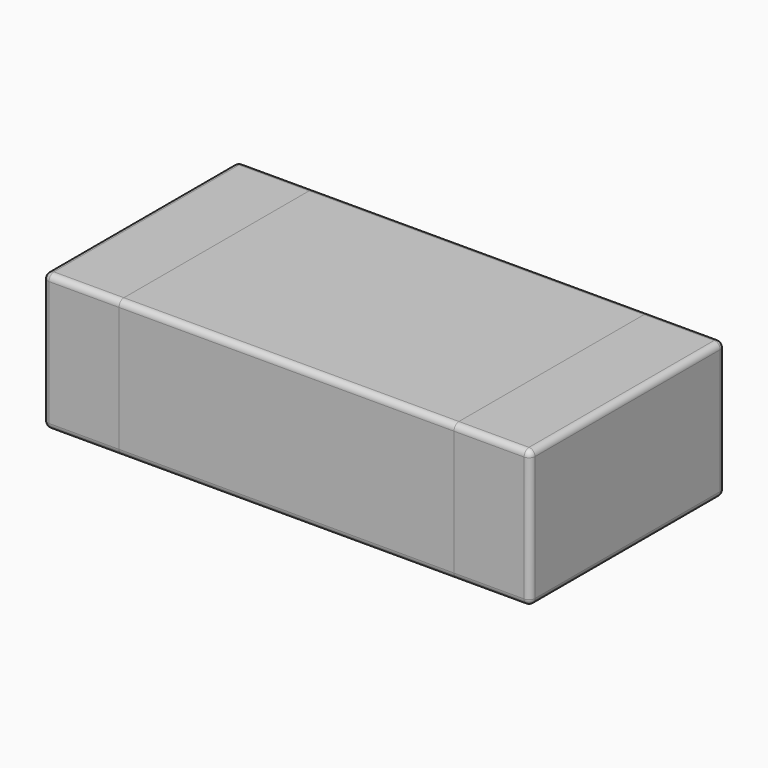
from build123d import *

# Parameters (mm, degrees)
F2_W     = 1.1
F2_H     = 0.8
F3_DEPTH = 0.43
F2_W_2   = 0.25
F4_DEPTH = 0.45
F5_DEPTH = 0.45
F6_DEPTH = 0.02
F7_R     = 0.01999
F7_2_R   = 0.01999
F7_3_R   = 0.01999
F7_4_R   = 0.01999


# Not quite as in the source:
# - a fillet or chamfer is up to 0.001 mm smaller than in the source, because OpenCascade refuses the exact size


with BuildPart() as f3:
    # F2 (on Top) → F3 (new body)
    with BuildSketch(Plane.XY):
        Rectangle(F2_W, F2_H)
    extrude(amount=F3_DEPTH)


with BuildPart() as f4:
    # F2 (on Top) → F4 (new body)
    with BuildSketch(Plane.XY):
        with Locations((-0.675, 0)):
            Rectangle(F2_W_2, F2_H)
    extrude(amount=F4_DEPTH)

    # F7 (radius 0.02 in the source; OpenCascade refuses exactly that, so slightly less here)
    f7_edges = [f4.edges().sort_by_distance(p)[0] for p in [
        (-0.675, -0.4, 0.45),
        (-0.8, 0.4, 0.225),
        (-0.8, -0.4, 0.225),
        (-0.8, 0, 0),
        (-0.8, 0, 0.45),
        (-0.675, 0.4, 0.45),
        (-0.675, 0.4, 0),
        (-0.675, -0.4, 0),
    ]]
    fillet(f7_edges, radius=F7_R)


with BuildPart() as f5:
    # F2 (on Top) → F5 (new body)
    with BuildSketch(Plane.XY):
        with Locations((0.675, 0)):
            Rectangle(F2_W_2, F2_H)
    extrude(amount=F5_DEPTH)

    # F7#2 (radius 0.02 in the source; OpenCascade refuses exactly that, so slightly less here)
    f7_2_edges = [f5.edges().sort_by_distance(p)[0] for p in [
        (0.675, -0.4, 0.45),
        (0.8, -0.4, 0.225),
        (0.8, 0.4, 0.225),
        (0.8, 0, 0),
        (0.8, 0, 0.45),
        (0.675, 0.4, 0.45),
        (0.675, 0.4, 0),
        (0.675, -0.4, 0),
    ]]
    fillet(f7_2_edges, radius=F7_2_R)


with BuildPart() as f6:
    # F6 (new): a face of the model
    f6_faces = [f3.part.faces().sort_by_distance(p)[0] for p in [
        (0, 0, 0.43),
    ]]
    extrude(f6_faces, amount=F6_DEPTH)

    # F7#4 (radius 0.02 in the source; OpenCascade refuses exactly that, so slightly less here)
    f7_4_edges = [f6.edges().sort_by_distance(p)[0] for p in [
        (0, -0.4, 0.45),
        (0, 0.4, 0.45),
    ]]
    fillet(f7_4_edges, radius=F7_4_R)


with BuildPart() as f3_1:
    add(f3.part)

    # F7#3 (radius 0.02 in the source; OpenCascade refuses exactly that, so slightly less here)
    f7_3_edges = [f3_1.edges().sort_by_distance(p)[0] for p in [
        (0, 0.4, 0),
        (0, -0.4, 0),
    ]]
    fillet(f7_3_edges, radius=F7_3_R)


solid = Compound([f4.part, f5.part, f6.part, f3_1.part])
